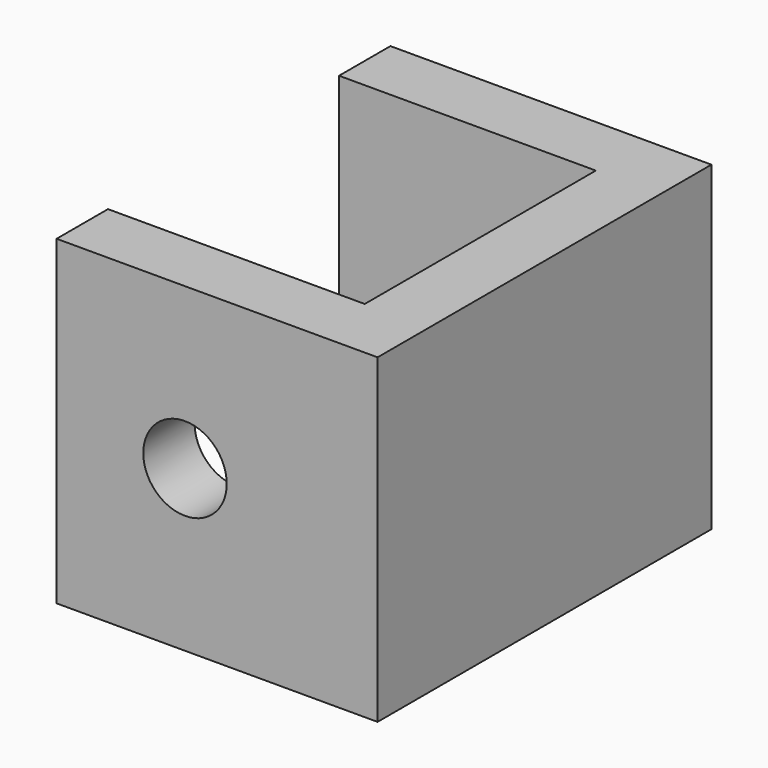
from build123d import *

# Parameters (mm, degrees)
F1_DEPTH = 10
F2_R     = 1.3
F3_DEPTH = 2


# Not quite as in the source:
# - a feature names something its author has since deleted; it is built from what else it names


with BuildPart() as f1:
    # F0 (on Top) → F1 (new body)
    with BuildSketch(Plane.XY):
        Polygon((-5, -6.5), (5, -6.5), (5, 6.5), (-5, 6.5), (-5, 4.5), (-3, 4.5), (3, 4.5), (3, -4.5), (-3, -4.5), (-5, -4.5), align=None)
    extrude(amount=F1_DEPTH)

    # F2 (on face) → F3 (cut, through all)
    with BuildSketch(Plane.XZ.offset(6.5)):
        with Locations((-1, 5)):
            Circle(F2_R)
    extrude(amount=-F3_DEPTH, mode=Mode.SUBTRACT)


solid = f1.part
